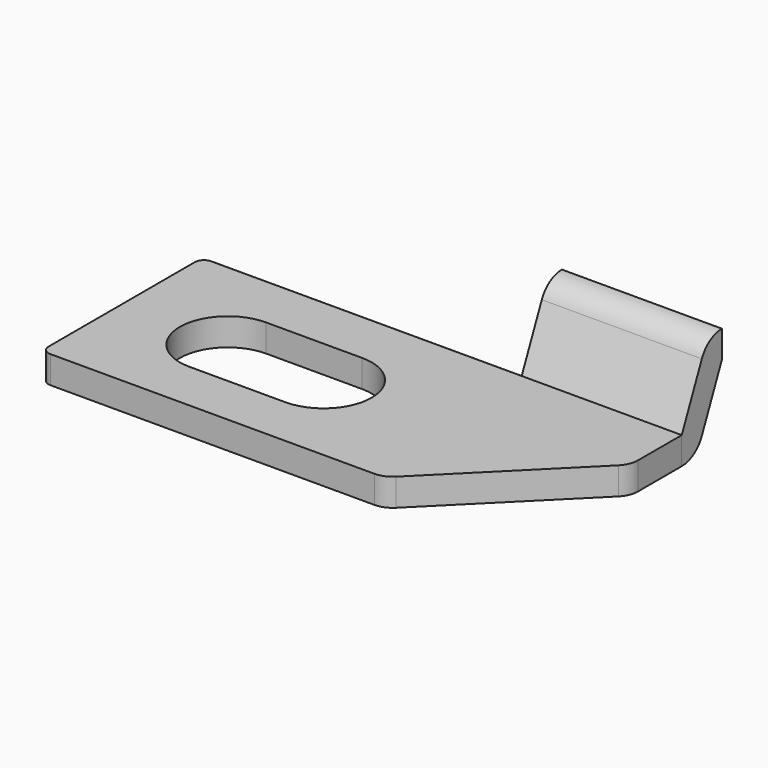
from build123d import *

# Parameters (mm, degrees)
F1_DEPTH = 50
F2_W     = 43.9973853057
F2_H     = 6
F3_DEPTH = 125


# Not quite as in the source:
# - ends of sketch curves that miss each other by under 0.0002 mm in the source are joined
# - a feature names something its author has since deleted; it is built from what else it names


with BuildPart() as f1:
    # F0 (on Top) → F1 (new body, symmetric)
    with BuildSketch(Plane.XY):
        Polygon((15.8618143265, -2.6014313847), (15.8618143265, -13.6014313847), (50.9007196128, -13.6014313847), (50.8959237908, -2.6014324301), align=None)
        with BuildLine():
            Line((15.8618143265, -13.6014313847), (-52.0992803872, -13.6014313847))
            ThreePointArc((-52.0992803872, -13.6014313847), (-53.5134939495, -14.1872178223), (-54.0992803872, -15.6014313847))
            Line((-54.0992803872, -15.6014313847), (-54.0992803872, -55.6014313847))
            ThreePointArc((-54.0992803872, -55.6014313847), (-53.5134939495, -57.0156449471), (-52.0992803872, -57.6014313847))
            Line((-52.0992803872, -57.6014313847), (18.8248942664, -57.6014313847))
            ThreePointArc((18.8248942664, -57.6014313847), (20.7365745268, -57.2215481129), (22.3577686464, -56.1396228175))
            Line((22.3577686464, -56.1396228175), (49.4335939928, -29.1044859403))
            ThreePointArc((49.4335939928, -29.1044859403), (50.5193975568, -27.4814483002), (50.9007196128, -25.5662945075))
            Line((50.9007196128, -25.5662945075), (50.9007196128, -13.6014313847))
            Line((50.9007196128, -13.6014313847), (15.8618143265, -13.6014313847))
        make_face()
        with BuildLine():
            ThreePointArc((-30.6326959729, -46.4203889966), (-41.1326959729, -35.9203889966), (-30.6326959729, -25.4203889966))
            Line((-30.6326959729, -25.4203889966), (-9.6326959729, -25.4203889966))
            ThreePointArc((-9.6326959729, -25.4203889966), (0.8673040271, -35.9203889966), (-9.6326959729, -46.4203889966))
            Line((-9.6326959729, -46.4203889966), (-30.6326959729, -46.4203889966))
        make_face(mode=Mode.SUBTRACT)
    extrude(amount=F1_DEPTH, both=True)


with BuildPart() as f3:
    # F2 (on Right) → F3 (new body, symmetric)
    with BuildSketch(Plane.YZ):
        Polygon((-2.610102063, 37.4432504177), (-2.610102063, 31.4432504177), (54.789897937, 31.4432504177), (54.7872818802, 37.4557568013), align=None)
        with BuildLine():
            Line((-8.1155181983, 18.9779470539), (-2.610102063, 31.4432504177))
            Line((-2.610102063, 31.4432504177), (-2.6127167571, 37.443249848))
            ThreePointArc((-2.6127167571, 37.443249848), (-5.8865329423, 36.4696806314), (-8.0986299437, 33.8673093492))
            Line((-8.0986299437, 33.8673093492), (-13.6040460789, 21.4020059854))
            Line((-13.6040460789, 21.4020059854), (-13.6040460789, 15.4020059854))
            ThreePointArc((-13.6040460789, 15.4020059854), (-10.3287104922, 16.3748619856), (-8.1155181983, 18.9779470539))
        make_face()
        Polygon((-2.6127167571, 37.443249848), (-2.610102063, 31.4432504177), (-2.610102063, 37.4432504177), align=None)
        with Locations((-35.6027387318, 18.4020059854)):
            Rectangle(F2_W, F2_H)
    extrude(amount=F3_DEPTH, both=True)

    # F4: intersect F1
    add(f1.part, mode=Mode.INTERSECT)


solid = f3.part
